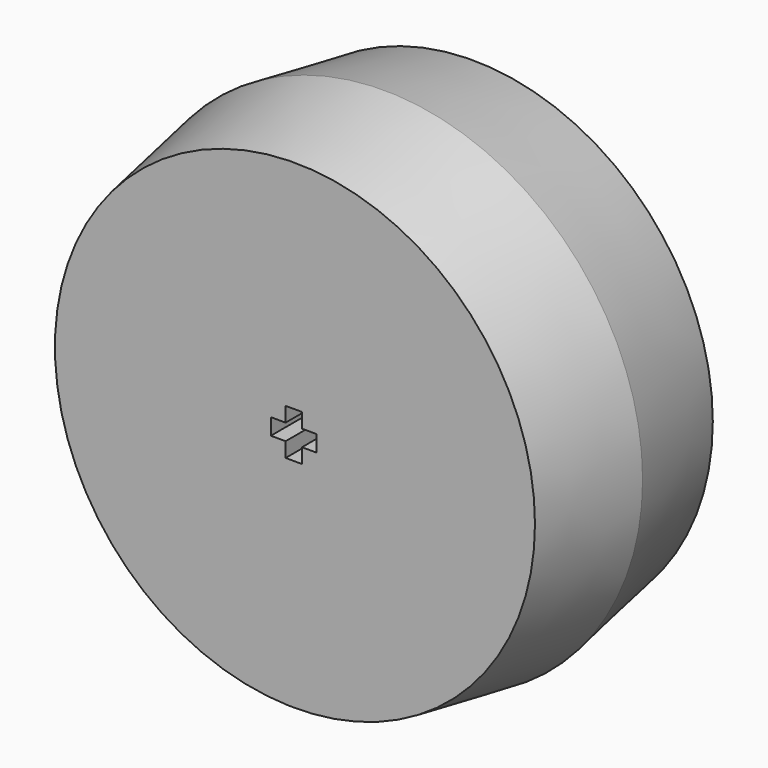
from build123d import *

# Parameters (mm, degrees)
F0_R       = 27.7
F1_DEPTH   = 23.8
F2_SIZE2   = 11.9
F2_SIZE    = 2
F2_2_SIZE2 = 11.89999
F2_2_SIZE  = 1.99999


# Not quite as in the source:
# - a fillet or chamfer is up to 0.001 mm smaller than in the source, because OpenCascade refuses the exact size


with BuildPart() as f1:
    # F0 (on Front) → F1 (new body)
    with BuildSketch(Plane.XZ):
        with Locations((0.358, -0.004)):
            Circle(F0_R)
        Polygon((-2.222, -0.874), (-2.222, -0.004), (-2.222, 0.876), (-0.642, 0.876), (-0.642, 2.456), (1.108, 2.456), (1.108, 0.876), (2.688, 0.876), (2.688, -0.874), (1.108, -0.874), (1.108, -2.454), (-0.642, -2.454), (-0.642, -0.874), align=None, mode=Mode.SUBTRACT)
    extrude(amount=F1_DEPTH)

    # F2
    f2_edges = [f1.edges().sort_by_distance(p)[0] for p in [
        (-27.342, -23.8, -0.004),
    ]]
    f2_side = f1.faces().sort_by_distance((-26.558526, -23.8, -0.004))[0]
    chamfer(f2_edges, length=F2_SIZE, length2=F2_SIZE2, reference=f2_side)

    # F2#2 (size 2 and 11.9 in the source; OpenCascade refuses exactly that, so slightly less here)
    f2_2_edges = [f1.edges().sort_by_distance(p)[0] for p in [
        (-27.342, 0, -0.004),
    ]]
    f2_2_side = f1.faces().sort_by_distance((-26.558526, 0, -0.004))[0]
    chamfer(f2_2_edges, length=F2_2_SIZE, length2=F2_2_SIZE2, reference=f2_2_side)


solid = f1.part
